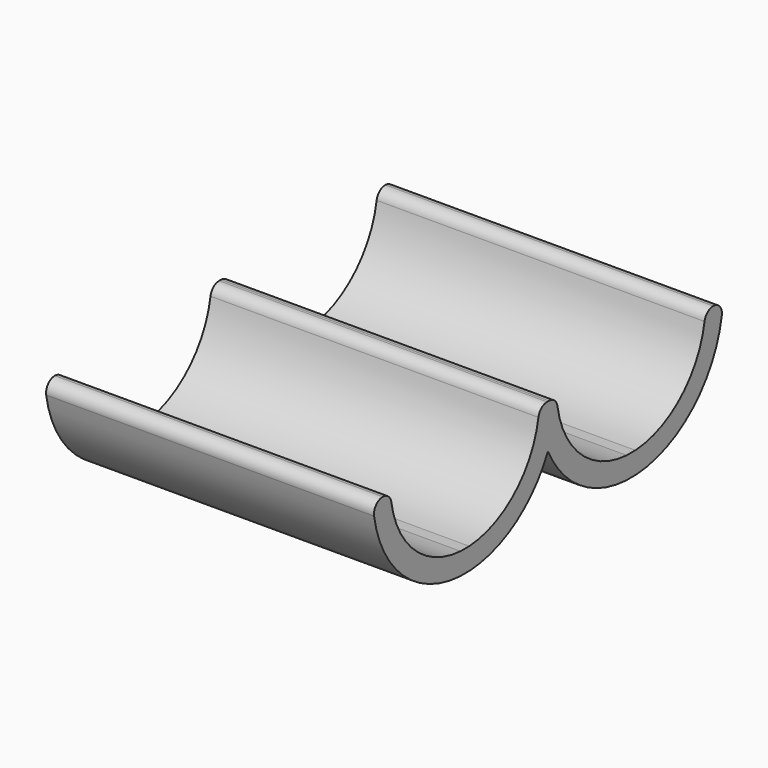
from build123d import *

# Parameters (mm, degrees)
F1_DEPTH = 30
F2_R     = 1
F3_R     = 0.9999
F4_R     = 0.99999


# Not quite as in the source:
# - a fillet or chamfer is up to 0.001 mm smaller than in the source, because OpenCascade refuses the exact size


with BuildPart() as f1:
    # F0 (on Right) → F1 (new body)
    with BuildSketch(Plane.YZ):
        with BuildLine():
            Line((0, 8), (-1, 8))
            Line((-1, 8), (-2, 8))
            ThreePointArc((-2, 8), (-4.4792027106, 2.4792027106), (-10, 0))
            Line((-10, 0), (-11, 0))
            ThreePointArc((-11, 0), (-16.5207972894, 2.4792027106), (-19, 8))
            Line((-19, 8), (-20.9965492395, 8))
            Line((-20.9965492395, 8), (-20.9965492395, 7.8825559271))
            ThreePointArc((-20.9965492395, 7.8825559271), (-17.9350112011, 1.0649887989), (-11.1174440729, -1.9965492395))
            Line((-11.1174440729, -1.9965492395), (-9.8825559561, -1.9965487463))
            ThreePointArc((-9.8825559561, -1.9965487463), (-4.6211597315, -0.2176837422), (-1, 3.9934744279))
            ThreePointArc((-1, 3.9934744279), (2.6211597315, -0.2176837422), (7.8825559561, -1.9965487463))
            Line((7.8825559561, -1.9965487463), (9.1174440439, -1.9965487463))
            ThreePointArc((9.1174440439, -1.9965487463), (15.9350108518, 1.0649891482), (18.9965487463, 7.8825559561))
            Line((18.9965487463, 7.8825559561), (18.9965487463, 8))
            Line((18.9965487463, 8), (17, 8))
            ThreePointArc((17, 8), (14.5207972894, 2.4792027106), (9, 0))
            Line((9, 0), (8, 0))
            ThreePointArc((8, 0), (2.4792027106, 2.4792027106), (0, 8))
        make_face()
    extrude(amount=F1_DEPTH)

    # F2
    f2_edges = [f1.edges().sort_by_distance(p)[0] for p in [
        (15, -19, 8),
    ]]
    fillet(f2_edges, radius=F2_R)

    # F3 (radius 1 in the source; OpenCascade refuses exactly that, so slightly less here)
    f3_edges = [f1.edges().sort_by_distance(p)[0] for p in [
        (15, -20.996549, 8),
    ]]
    fillet(f3_edges, radius=F3_R)

    # F4 (radius 1 in the source; OpenCascade refuses exactly that, so slightly less here)
    f4_edges = [f1.edges().sort_by_distance(p)[0] for p in [
        (15, -2, 8),
        (15, 0, 8),
        (15, 18.996549, 8),
        (15, 17, 8),
    ]]
    fillet(f4_edges, radius=F4_R)


solid = f1.part
